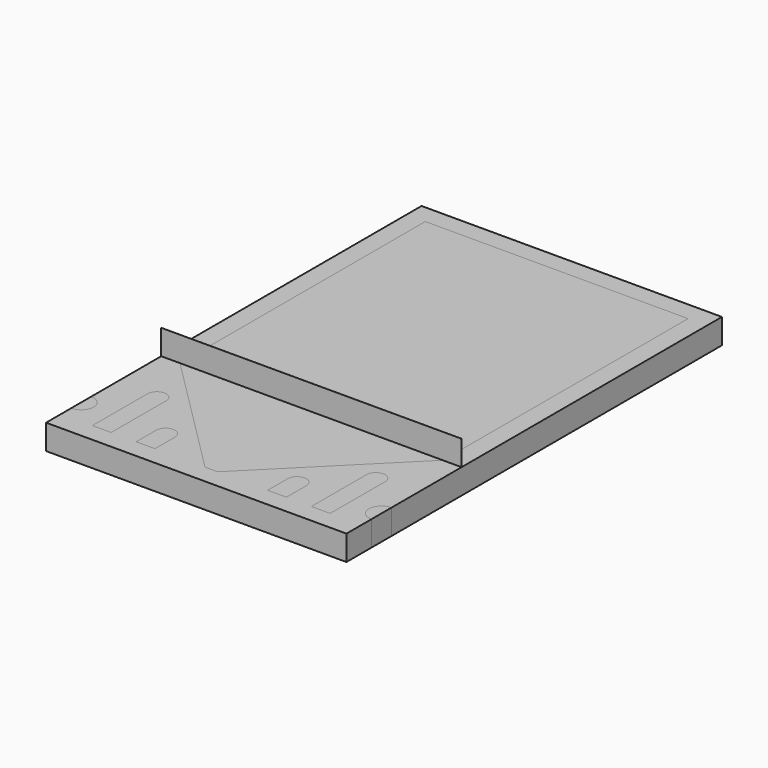
from build123d import *

# Parameters (mm, degrees)
F0_W      = 152.4
F0_H      = 238.125
F1_DEPTH  = 12.7
F3_DEPTH  = 12.7
F5_DEPTH  = 25.4
F7_DEPTH  = 12.7
F9_DEPTH  = 12.7
F11_E36_W = 152.4
F11_E36_H = 12.7
F12_DEPTH = 0.0127


with BuildPart() as f1:
    # F0 (on Top) → F1 (new body)
    with BuildSketch(Plane.XY):
        with Locations((76.2, -119.0625)):
            Rectangle(F0_W, F0_H)
        Polygon((9.525, -9.525), (142.875, -9.525), (142.875, -165.1), (79.375, -228.6), (73.025, -228.6), (9.525, -165.1), align=None, mode=Mode.SUBTRACT)
    extrude(amount=F1_DEPTH)

    # F2 (on face) → F3 (cut, through all)
    with BuildSketch(Plane.XY.offset(12.7)):
        with BuildLine():
            Line((0, -209.55), (0, -222.25))
            ThreePointArc((0, -222.25), (6.35, -215.9), (0, -209.55))
        make_face()
        with BuildLine():
            ThreePointArc((152.4, -209.55), (146.05, -215.9), (152.4, -222.25))
            Line((152.4, -222.25), (152.4, -209.55))
        make_face()
    extrude(amount=-F3_DEPTH, mode=Mode.SUBTRACT)

    # F4 (on face) → F5 (cut)
    with BuildSketch(Plane.XY.offset(12.7)):
        with BuildLine():
            Line((15.875, -193.675), (15.875, -228.6))
            Line((15.875, -228.6), (25.4, -228.6))
            Line((25.4, -228.6), (25.4, -193.675))
            ThreePointArc((25.4, -193.675), (20.6375, -188.9125), (15.875, -193.675))
        make_face()
        with BuildLine():
            Line((38.1, -215.9), (38.1, -228.6))
            Line((38.1, -228.6), (47.625, -228.6))
            Line((47.625, -228.6), (47.625, -215.9))
            ThreePointArc((47.625, -215.9), (42.8625, -211.1375), (38.1, -215.9))
        make_face()
        with BuildLine():
            ThreePointArc((136.525, -193.675), (131.7625, -188.9125), (127, -193.675))
            Line((127, -193.675), (127, -228.6))
            Line((127, -228.6), (136.525, -228.6))
            Line((136.525, -228.6), (136.525, -193.675))
        make_face()
        with BuildLine():
            Line((104.775, -215.9), (104.775, -228.6))
            Line((104.775, -228.6), (114.3, -228.6))
            Line((114.3, -228.6), (114.3, -215.9))
            ThreePointArc((114.3, -215.9), (109.5375, -211.1375), (104.775, -215.9))
        make_face()
    extrude(amount=-F5_DEPTH, mode=Mode.SUBTRACT)


with BuildPart() as f7:
    # F6 (on face) → F7 (new body)
    with BuildSketch(Plane.XY.offset(12.7)):
        Polygon((9.525, -9.525), (9.525, -165.1), (73.025, -228.6), (79.375, -228.6), (142.875, -165.1), (142.875, -9.525), align=None)
    extrude(amount=-F7_DEPTH)


with BuildPart() as f7b:
    # F6 (on face) → F7, piece 2 (new body)
    with BuildSketch(Plane.XY.offset(12.7)):
        with BuildLine():
            Line((15.875, -193.675), (15.875, -228.6))
            Line((15.875, -228.6), (25.4, -228.6))
            Line((25.4, -228.6), (25.4, -193.675))
            ThreePointArc((25.4, -193.675), (20.6375, -188.9125), (15.875, -193.675))
        make_face()
    extrude(amount=-F7_DEPTH)


with BuildPart() as f7c:
    # F6 (on face) → F7, piece 3 (new body)
    with BuildSketch(Plane.XY.offset(12.7)):
        with BuildLine():
            Line((47.625, -228.6), (47.625, -215.9))
            ThreePointArc((47.625, -215.9), (42.8625, -211.1375), (38.1, -215.9))
            Line((38.1, -215.9), (38.1, -228.6))
            Line((38.1, -228.6), (47.625, -228.6))
        make_face()
    extrude(amount=-F7_DEPTH)


with BuildPart() as f7d:
    # F6 (on face) → F7, piece 4 (new body)
    with BuildSketch(Plane.XY.offset(12.7)):
        with BuildLine():
            Line((104.775, -215.9), (104.775, -228.6))
            Line((104.775, -228.6), (114.3, -228.6))
            Line((114.3, -228.6), (114.3, -215.9))
            ThreePointArc((114.3, -215.9), (109.5375, -211.1375), (104.775, -215.9))
        make_face()
    extrude(amount=-F7_DEPTH)


with BuildPart() as f7e:
    # F6 (on face) → F7, piece 5 (new body)
    with BuildSketch(Plane.XY.offset(12.7)):
        with BuildLine():
            ThreePointArc((136.525, -193.675), (131.7625, -188.9125), (127, -193.675))
            Line((127, -193.675), (127, -228.6))
            Line((127, -228.6), (136.525, -228.6))
            Line((136.525, -228.6), (136.525, -193.675))
        make_face()
    extrude(amount=-F7_DEPTH)


with BuildPart() as f9:
    # F8 (on face) → F9 (new body)
    with BuildSketch(Plane.XY.offset(12.7)):
        with BuildLine():
            Line((0, -209.55), (0, -222.25))
            ThreePointArc((0, -222.25), (6.35, -215.9), (0, -209.55))
        make_face()
    extrude(amount=-F9_DEPTH)


with BuildPart() as f9b:
    # F8 (on face) → F9, piece 2 (new body)
    with BuildSketch(Plane.XY.offset(12.7)):
        with BuildLine():
            Line((152.4, -222.25), (152.4, -209.55))
            ThreePointArc((152.4, -209.55), (146.05, -215.9), (152.4, -222.25))
        make_face()
    extrude(amount=-F9_DEPTH)


with BuildPart() as f12:
    # F11_E36 (on explicit) → F12 (new body)
    with BuildSketch(Plane(origin=(0, -165.1, 12.7), x_dir=(1, 0, 0), z_dir=(0, -1, 0))):
        with Locations((76.2, 6.35)):
            Rectangle(F11_E36_W, F11_E36_H)
    extrude(amount=F12_DEPTH)


solid = Compound([f1.part, f7.part, f7b.part, f7c.part, f7d.part, f7e.part, f9.part, f9b.part, f12.part])
